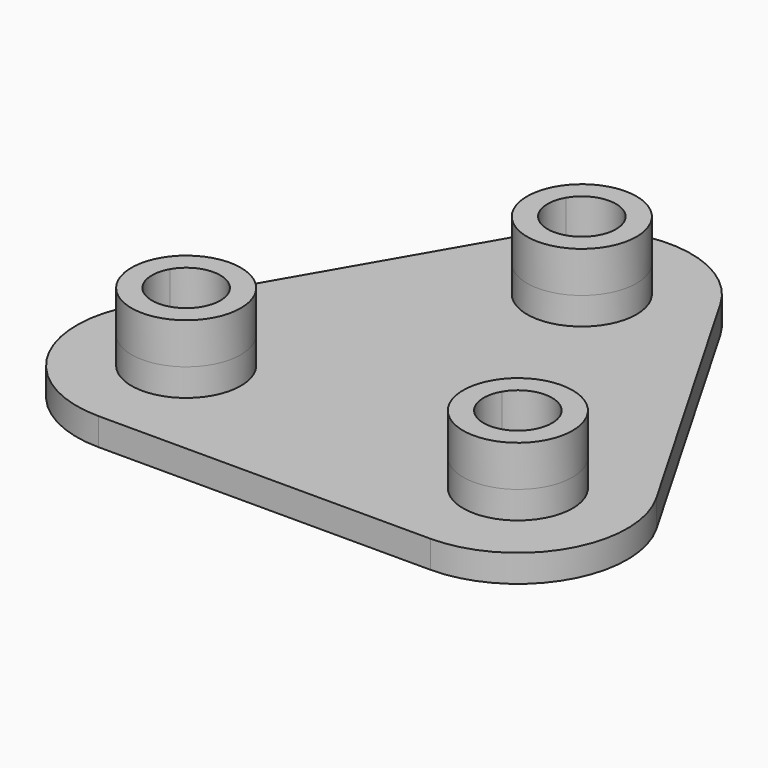
from build123d import *

# Parameters (mm, degrees)
F1_DEPTH = 6.35
F2_R     = 7.9375
F2_R_2   = 3.175
F3_DEPTH = 6.35
F4_R     = 12.7
F5_DEPTH = 6.35
F6_DEPTH = 9.525


with BuildPart() as f1:
    # F0 (on Top) → F1 (new body)
    with BuildSketch(Plane.XY):
        with BuildLine():
            Line((-31.6207525557, -18.25625), (0, 0))
            Line((0, 0), (0, 36.5125))
            ThreePointArc((0, 36.5125), (-6.8740766425, 40.48125), (-6.8740766425, 48.41875))
            Line((-6.8740766425, 48.41875), (-21.9970452561, 57.15))
            Line((-21.9970452561, 57.15), (-60.4918744543, -9.525))
            Line((-60.4918744543, -9.525), (-45.3689058408, -18.25625))
            ThreePointArc((-45.3689058408, -18.25625), (-38.4948291982, -14.2875), (-31.6207525557, -18.25625))
        make_face()
        with BuildLine():
            ThreePointArc((-38.4948291982, -30.1625), (-45.3689058408, -26.19375), (-45.3689058408, -18.25625))
            Line((-45.3689058408, -18.25625), (-60.4918744543, -9.525))
            ThreePointArc((-60.4918744543, -9.525), (-60.4918744543, -34.925), (-38.4948291982, -47.625))
            Line((-38.4948291982, -47.625), (-38.4948291982, -30.1625))
        make_face()
        with BuildLine():
            Line((31.6207525557, -18.25625), (0, 0))
            Line((0, 0), (-31.6207525557, -18.25625))
            ThreePointArc((-31.6207525557, -18.25625), (-30.827792952, -20.1706238295), (-30.5573291982, -22.225))
            ThreePointArc((-30.5573291982, -22.225), (-32.8821691226, -27.8376600757), (-38.4948291982, -30.1625))
            Line((-38.4948291982, -30.1625), (-38.4948291982, -47.625))
            Line((-38.4948291982, -47.625), (38.4948291982, -47.625))
            Line((38.4948291982, -47.625), (38.4948291982, -30.1625))
            ThreePointArc((38.4948291982, -30.1625), (31.6207525557, -26.19375), (31.6207525557, -18.25625))
        make_face()
        with BuildLine():
            Line((60.4918744543, -9.525), (45.3689058408, -18.25625))
            ThreePointArc((45.3689058408, -18.25625), (46.1618654444, -20.1706238295), (46.4323291982, -22.225))
            ThreePointArc((46.4323291982, -22.225), (44.1074892739, -27.8376600757), (38.4948291982, -30.1625))
            Line((38.4948291982, -30.1625), (38.4948291982, -47.625))
            ThreePointArc((38.4948291982, -47.625), (60.4918744543, -34.925), (60.4918744543, -9.525))
        make_face()
        with BuildLine():
            Line((0, 36.5125), (0, 0))
            Line((0, 0), (31.6207525557, -18.25625))
            ThreePointArc((31.6207525557, -18.25625), (38.4948291982, -14.2875), (45.3689058408, -18.25625))
            Line((45.3689058408, -18.25625), (60.4918744543, -9.525))
            Line((60.4918744543, -9.525), (21.9970452561, 57.15))
            Line((21.9970452561, 57.15), (6.8740766425, 48.41875))
            ThreePointArc((6.8740766425, 48.41875), (7.6670362462, 46.5043761705), (7.9375, 44.45))
            ThreePointArc((7.9375, 44.45), (5.6126600757, 38.8373399243), (0, 36.5125))
        make_face()
        with BuildLine():
            Line((-21.9970452561, 57.15), (-6.8740766425, 48.41875))
            ThreePointArc((-6.8740766425, 48.41875), (0, 52.3875), (6.8740766425, 48.41875))
            Line((6.8740766425, 48.41875), (21.9970452561, 57.15))
            ThreePointArc((21.9970452561, 57.15), (0, 69.85), (-21.9970452561, 57.15))
        make_face()
    extrude(amount=F1_DEPTH)

    # F2 (on face) → F3 (join)
    with BuildSketch(Plane(origin=(0, 0, 0), x_dir=(1, 0, 0), z_dir=(0, 0, -1))):
        with BuildLine():
            ThreePointArc((-38.4948291982, 47.625), (-60.4918744543, 34.925), (-60.4918744543, 9.525))
            Line((-60.4918744543, 9.525), (-21.9970452561, -57.15))
            ThreePointArc((-21.9970452561, -57.15), (0, -69.85), (21.9970452561, -57.15))
            Line((21.9970452561, -57.15), (60.4918744543, 9.525))
            ThreePointArc((60.4918744543, 9.525), (60.4918744543, 34.925), (38.4948291982, 47.625))
            Line((38.4948291982, 47.625), (-38.4948291982, 47.625))
        make_face()
        with Locations((0, -44.45)):
            Circle(F2_R, mode=Mode.SUBTRACT)
        with Locations((-38.4948291982, 22.225)):
            Circle(F2_R, mode=Mode.SUBTRACT)
        with Locations((38.4948291982, 22.225)):
            Circle(F2_R, mode=Mode.SUBTRACT)
        with Locations((0, -44.45)):
            Circle(F2_R)
        with Locations((0, -44.45)):
            Circle(F2_R_2, mode=Mode.SUBTRACT)
        with Locations((38.4948291982, 22.225)):
            Circle(F2_R)
        with Locations((38.4948291982, 22.225)):
            Circle(F2_R_2, mode=Mode.SUBTRACT)
        with Locations((-38.4948291982, 22.225)):
            Circle(F2_R)
        with Locations((-38.4948291982, 22.225)):
            Circle(F2_R_2, mode=Mode.SUBTRACT)
    extrude(amount=F3_DEPTH)

    # F4 (on face) → F5 (cut)
    with BuildSketch(Plane.XY.offset(6.35)):
        with BuildLine():
            ThreePointArc((21.9970452561, 57.15), (0, 69.85), (-21.9970452561, 57.15))
            Line((-21.9970452561, 57.15), (-60.4918744543, -9.525))
            ThreePointArc((-60.4918744543, -9.525), (-60.4918744543, -34.925), (-38.4948291982, -47.625))
            Line((-38.4948291982, -47.625), (38.4948291982, -47.625))
            ThreePointArc((38.4948291982, -47.625), (60.4918744543, -34.925), (60.4918744543, -9.525))
            Line((60.4918744543, -9.525), (21.9970452561, 57.15))
        make_face()
        with Locations((-38.4948291982, -22.225)):
            Circle(F4_R, mode=Mode.SUBTRACT)
        with Locations((38.4948291982, -22.225)):
            Circle(F4_R, mode=Mode.SUBTRACT)
        with Locations((0, 44.45)):
            Circle(F4_R, mode=Mode.SUBTRACT)
    extrude(amount=-F5_DEPTH, mode=Mode.SUBTRACT)

    # F6 (add): faces of the model
    f6_faces = [f1.faces().sort_by_distance(p)[0] for p in [
        (-50.8356189534, -22.225, 6.35),
        (-12.3407897552, 44.45, 6.35),
        (26.1540394431, -22.225, 6.35),
    ]]
    extrude(f6_faces, amount=F6_DEPTH)


solid = f1.part
